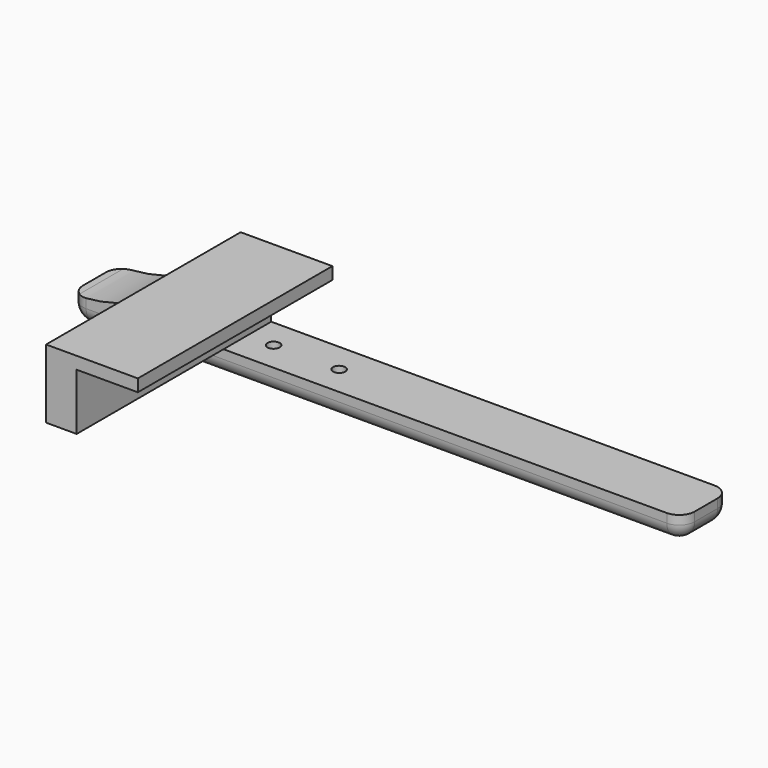
from build123d import *

# Parameters (mm, degrees)
F0_W            = 200
F0_H            = 19.5
F1_DEPTH        = 8
F2_W            = 10
F2_H            = 19.5
F3_DEPTH        = 22.5
F4_W            = 19.5
F4_H            = 4
F5_DEPTH        = 20
F7_DEPTH        = 60
F9_D            = 4
F9_DEPTH        = 8
F9_CSINK_D      = 8
F9_CSINK_ANGLE  = 82
F9_TIP          = 1.2017212381
F10_T1_DEPTH    = 19.5
F12_D           = 5
F12_DEPTH       = 20
F12_CSINK_D     = 9.5
F12_CSINK_ANGLE = 82
F12_TIP         = 1.5021515476
F13_R           = 5.08


# Not quite as in the source:
# - a fillet or chamfer that OpenCascade refuses, or shapes differently, is made with other operations: its cross-section is extruded or revolved along the edge and cut away or added


with BuildPart() as f1:
    # F0 (on Top) → F1 (new body)
    with BuildSketch(Plane.XY):
        with Locations((76.8052995205, 5.1813468188)):
            Rectangle(F0_W, F0_H)
    extrude(amount=F1_DEPTH)

    # F2 (on face) → F3 (join)
    with BuildSketch(Plane.XY.offset(8)):
        with Locations((21.8052995205, 5.1813468188)):
            Rectangle(F2_W, F2_H)
    extrude(amount=F3_DEPTH)

    # F4 (on face) → F5 (join)
    with BuildSketch(Plane.YZ.offset(26.8052995205)):
        with Locations((5.1813468188, 28.5)):
            Rectangle(F4_W, F4_H)
    extrude(amount=F5_DEPTH)

    # F6 (on face) → F7 (join)
    with BuildSketch(Plane.XZ.offset(4.5686531812)):
        Polygon((16.8052995205, 30.5), (16.8052995205, 8), (26.8052995205, 8), (26.8052995205, 26.5), (46.8052995205, 26.5), (46.8052995205, 30.5), align=None)
    extrude(amount=F7_DEPTH)

    # F9
    with Locations(Plane(origin=(0, 0, 0), x_dir=(1, 0, 0), z_dir=(0, 0, -1))):
        with Locations((35.3978276253, -5.1813468188), (56.8052995205, -5.1813468188)):
            CounterSinkHole(F9_D / 2, F9_CSINK_D / 2, depth=F9_DEPTH, counter_sink_angle=F9_CSINK_ANGLE)
            with Locations((0, 0, -(F9_DEPTH + F9_TIP / 2))):  # 118° drill point
                Cone(0, F9_D / 2, F9_TIP, mode=Mode.SUBTRACT)

    # F10: fillet of radius 42.924717139 on 1 edges, made by hand

    # F10_s2 → F10_t1 (join)
    with BuildSketch(Plane.XZ.offset(-14.9313468188)):
        with BuildLine():
            ThreePointArc((16.8052995205, 30.5), (1.0263848307, 14.0515795772), (-20.9486707509, 8))
            Line((-20.9486707509, 8), (16.8052995205, 8))
            Line((16.8052995205, 8), (16.8052995205, 30.5))
        make_face()
    extrude(amount=F10_T1_DEPTH)

    # F12
    with Locations(Plane(origin=(16.8052995205, 0, 0), x_dir=(0, -1, 0), z_dir=(-1, 0, 0))):
        with Locations((24.8886531812, 19.25), (45.2086531812, 19.25)):
            CounterSinkHole(F12_D / 2, F12_CSINK_D / 2, depth=F12_DEPTH, counter_sink_angle=F12_CSINK_ANGLE)
            with Locations((0, 0, -(F12_DEPTH + F12_TIP / 2))):  # 118° drill point
                Cone(0, F12_D / 2, F12_TIP, mode=Mode.SUBTRACT)

    # F13
    f13_edges = [f1.edges().sort_by_distance(p)[0] for p in [
        (76.8053, -4.568653, 0),
        (176.8053, 5.181347, 0),
        (76.8053, 14.931347, 0),
        (-23.1947, 5.181347, 0),
        (176.8053, 14.931347, 4),
        (176.8053, -4.568653, 4),
        (-23.1947, 14.931347, 4),
        (-23.1947, -4.568653, 4),
    ]]
    fillet(f13_edges, radius=F13_R)


solid = f1.part
